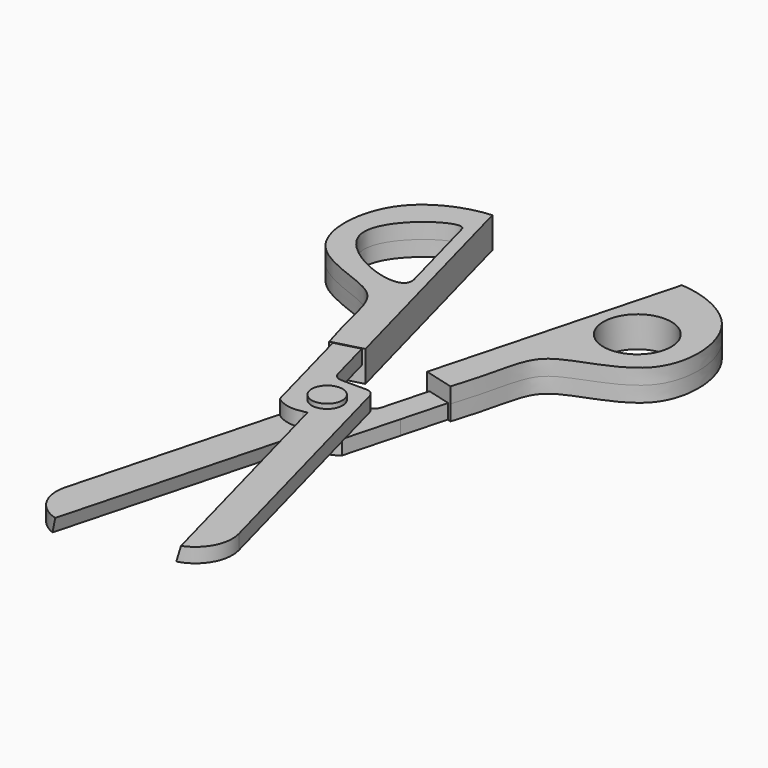
from build123d import *

# Parameters (mm, degrees)
F1_DEPTH  = 5
F3_DEPTH  = 20
F4_R      = 11
F5_DEPTH  = 20
F6_R      = 4
F7_DEPTH  = 6
F10_DEPTH = 2.35
F15_DEPTH = 80
F16_DEPTH = 2.35
F18_R     = 5
F19_DEPTH = 0.75
F22_DEPTH = 80
F24_R     = 5
F25_DEPTH = 0.75


# Not quite as in the source:
# - ends of sketch curves that miss each other by under 0.0002 mm in the source are joined


with BuildPart() as f1:
    # F0 (on Top) → F1 (new body, symmetric)
    with BuildSketch(Plane.XY):
        with BuildLine():
            Line((30.7055236082, 87.2740661031), (10, 10))
            Line((10, 10), (19.6592582629, 7.411809549))
            add(Edge.make_bspline(
                [(19.6592582629, 7.411809549), (25.1119283769, 24.3706590227), (23.1415058885, 37.2634909185), (60.0169233832, 42.5553149198), (57.5790190448, 80.8229242309), (36.3791040972, 87.095948963), (30.7055236082, 87.2740661031)],
                knots=[0, 0, 0, 0, 0.26106387, 0.5078740317, 0.7657061692, 1, 1, 1, 1], degree=3))
        make_face()
    extrude(amount=F1_DEPTH, both=True)

    # F4 (on Top) → F5 (cut, symmetric)
    with BuildSketch(Plane.XY):
        with Locations((38.723934875, 59.2436347694)):
            Circle(F4_R)
    extrude(amount=F5_DEPTH, both=True, mode=Mode.SUBTRACT)


with BuildPart() as f1b:
    # F0 (on Top) → F1, piece 2 (new body, symmetric)
    with BuildSketch(Plane.XY):
        with BuildLine():
            Line((-19.6592582629, 7.411809549), (-10, 10))
            Line((-10, 10), (-30.7055236082, 87.2740661031))
            add(Edge.make_bspline(
                [(-19.6592582629, 7.411809549), (-25.1119283769, 24.3706590227), (-23.1415058885, 37.2634909185), (-60.0169233832, 42.5553149198), (-57.5790190448, 80.8229242309), (-36.3791040972, 87.095948963), (-30.7055236082, 87.2740661031)],
                knots=[0, 0, 0, 0, 0.26106387, 0.5078740317, 0.7657061692, 1, 1, 1, 1], degree=3))
        make_face()
    extrude(amount=F1_DEPTH, both=True)

    # F2 (on Top) → F3 (cut, symmetric)
    with BuildSketch(Plane.XY):
        with BuildLine():
            Line((-24.2164651093, 47.6017568712), (-31.9810364623, 76.5795316598))
            add(Edge.make_bspline(
                [(-31.9810364623, 76.5795316598), (-33.2751316878, 81.4091607913), (-72.673683141, 55.6837191887), (-21.6282746582, 37.9424986083), (-24.2164651093, 47.6017568712)],
                knots=[0, 0, 0, 0, 0.4904361098, 1, 1, 1, 1], degree=3))
        make_face()
    extrude(amount=F3_DEPTH, both=True, mode=Mode.SUBTRACT)


with BuildPart() as f7:
    # F6 (on Top) → F7 (new body, symmetric)
    with BuildSketch(Plane.XY):
        with Locations((0, -18)):
            Circle(F6_R)
    extrude(amount=F7_DEPTH, both=True)

    # F18 (on offset) → F19 (join, symmetric)
    with BuildSketch(Plane.XY.offset(5.85)):
        with Locations((0, -18)):
            Circle(F18_R)
    extrude(amount=F19_DEPTH, both=True)

    # F24 (on offset) → F25 (join, symmetric)
    with BuildSketch(Plane(origin=(0, 0, -5.85), x_dir=(1, 0, 0), z_dir=(0, 0, -1))):
        with Locations((0, 18)):
            Circle(F24_R)
    extrude(amount=F25_DEPTH, both=True)


with BuildPart() as f10:
    # F9 (on offset) → F10 (new body, symmetric)
    with BuildSketch(Plane.XY.offset(2.5)):
        with BuildLine():
            Line((-12.2600210518, 14.5708100863), (-19.9874276621, 12.5002577255))
            Line((-19.9874276621, 12.5002577255), (-14.8110467601, -6.8182588003))
            Line((-14.8110467601, -6.8182588003), (-10.0427421803, -24.613813758))
            ThreePointArc((-10.0427421803, -24.613813758), (-5.7772962336, -26.5637923126), (-1.0919279377, -26.3545808891))
            Line((-1.0919279377, -26.3545808891), (19.6135956705, -103.6286469922))
            ThreePointArc((19.6135956705, -103.6286469922), (26.9000719747, -98.0375370768), (28.0988770448, -88.9317085355))
            Line((28.0988770448, -88.9317085355), (6.7277586225, -9.1736087692))
            ThreePointArc((6.7277586225, -9.1736087692), (5.7944584368, -7.6827262818), (4.1858626709, -6.9712493041))
            Line((4.1858626709, -6.9712493041), (0, -6.9712493041))
            Line((0, -6.9712493041), (-4.1858626709, -6.9712493041))
            ThreePointArc((-4.1858626709, -6.9712493041), (-6.0121469579, -6.351309325), (-7.0836401498, -4.7477064394))
            Line((-7.0836401498, -4.7477064394), (-12.2600210518, 14.5708100863))
        make_face()
    extrude(amount=F10_DEPTH, both=True)

    # F14 (on offset) → F15 (cut)
    with BuildSketch(Plane(origin=(27.2413648185, -101.66615757, 0), x_dir=(-0.9659258263, -0.2588190451, 0), z_dir=(-0.2588190451, 0.9659258263, 0))):
        Polygon((6.6164276508, 4.85), (7.8757888552, 0.15), (7.8757888552, 4.85), align=None)
    extrude(amount=F15_DEPTH, mode=Mode.SUBTRACT)

    # F27: cut F1b
    add(f1b.part, mode=Mode.SUBTRACT)

    # F28: cut F7
    add(f7.part, mode=Mode.SUBTRACT)


with BuildPart() as f16:
    # F12 (on offset) → F16 (new body, symmetric)
    with BuildSketch(Plane.XY.offset(-2.5)):
        with BuildLine():
            Line((19.9874276621, 12.5002577255), (12.2600210518, 14.5708100863))
            Line((12.2600210518, 14.5708100863), (7.0836401498, -4.7477064394))
            ThreePointArc((7.0836401498, -4.7477064394), (6.0122017645, -6.3512678388), (4.186, -6.9712494484))
            Line((4.186, -6.9712494484), (0, -6.9712494484))
            Line((0, -6.9712494484), (-4.186, -6.9712494484))
            ThreePointArc((-4.186, -6.9712494484), (-5.7945173505, -7.6827530429), (-6.7277693578, -9.1735937864))
            Line((-6.7277693578, -9.1735937864), (-28.0988907345, -88.9317045793))
            ThreePointArc((-28.0988907345, -88.9317045793), (-26.9000856645, -98.0375331205), (-19.6136093603, -103.628643036))
            Line((-19.6136093603, -103.628643036), (1.0919142479, -26.3545769328))
            ThreePointArc((1.0919142479, -26.3545769328), (5.7772892396, -26.5637936728), (10.0427421803, -24.613813758))
            Line((10.0427421803, -24.613813758), (14.8110467601, -6.8182588003))
            Line((14.8110467601, -6.8182588003), (19.9874276621, 12.5002577255))
        make_face()
    extrude(amount=F16_DEPTH, both=True)

    # F21 (on offset) → F22 (cut)
    with BuildSketch(Plane(origin=(-27.2413648185, -101.66615757, 0), x_dir=(-0.9659258263, 0.2588190451, 0), z_dir=(0.2588190451, 0.9659258263, 0))):
        Polygon((-6.6164134035, -4.85), (-7.875774608, -0.15), (-7.875774608, -4.85), align=None)
    extrude(amount=F22_DEPTH, mode=Mode.SUBTRACT)

    # F26: cut F1
    add(f1.part, mode=Mode.SUBTRACT)

    # F28: cut F7
    add(f7.part, mode=Mode.SUBTRACT)


solid = Compound([f1.part, f1b.part, f7.part, f10.part, f16.part])
